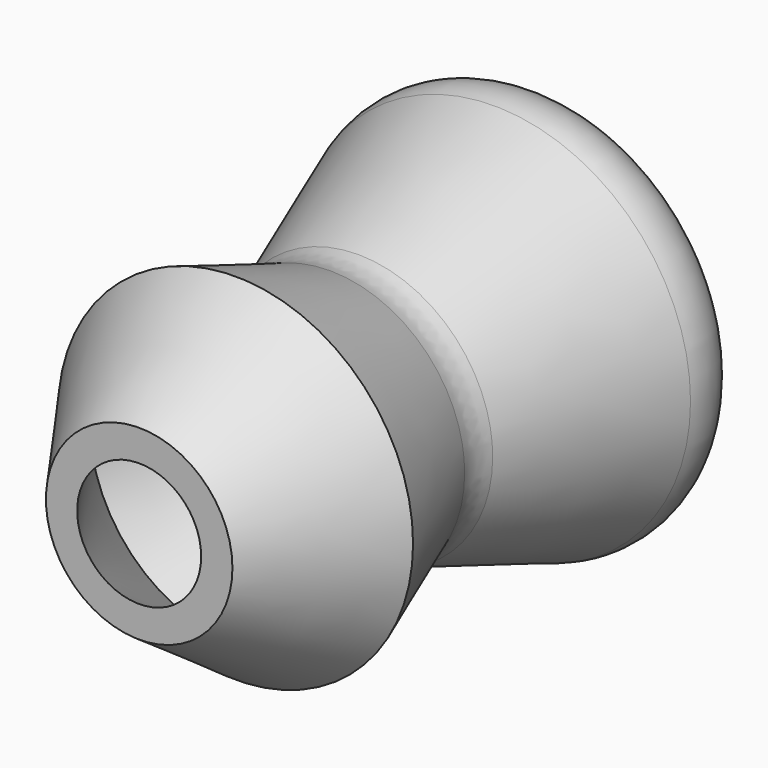
from build123d import *

# Parameters (mm, degrees)
F0_R     = 63.5
F1_DEPTH = 127
F1_TAPER = -20
F2_R     = 25.4
F4_T     = -12.7


# Not quite as in the source:
# - a fillet or chamfer that OpenCascade refuses, or shapes differently, is made with other operations: its cross-section is extruded or revolved along the edge and cut away or added


with BuildPart() as f1:
    # F0 (on Front) → F1 (new body, symmetric)
    with BuildSketch(Plane.XZ):
        Circle(F0_R)
    extrude(amount=F1_DEPTH, both=True, taper=F1_TAPER)

    # F2
    f2_edges = [f1.edges().sort_by_distance(p)[0] for p in [
        (-63.5, 0, 0),
        (-109.72422, 127, 0),
    ]]
    fillet(f2_edges, radius=F2_R)

    # F3: chamfer of 63.5 on 1 edges, made by hand

    # F3_s1 → F3_t2 (revolve, cut)
    with BuildSketch(Plane.XY):
        Polygon((88.0059406506, -67.3295185801), (46.2242197518, -127), (109.7242197518, -127), align=None)
    revolve(axis=Axis((0, -127, 0), (0, 1, 0)), mode=Mode.SUBTRACT)

    # F4
    f4_openings = [f1.faces().sort_by_distance(p)[0] for p in [
        (0, -127, 0),
    ]]
    offset(amount=F4_T, openings=f4_openings)


solid = f1.part
